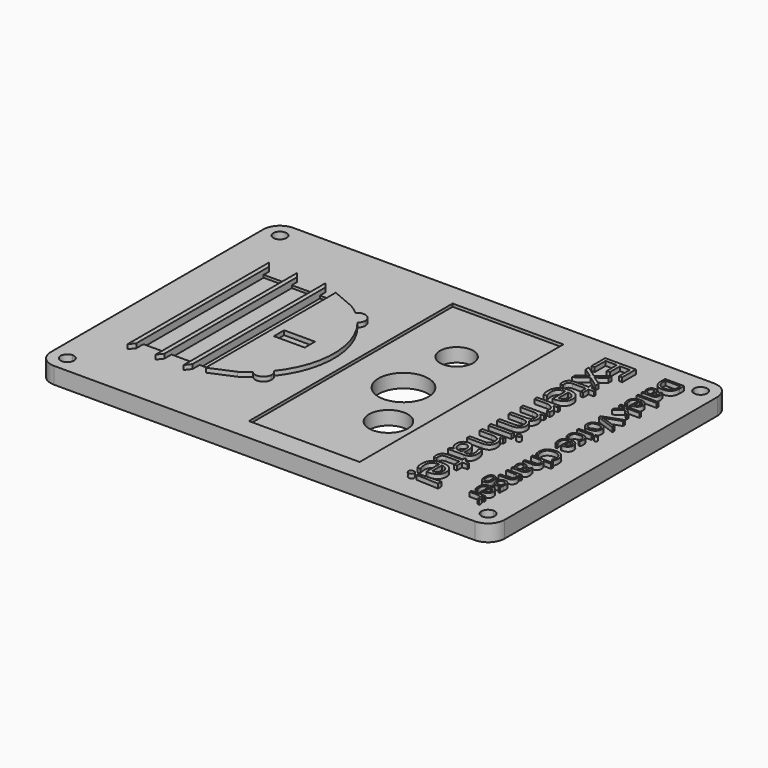
from build123d import *

# Parameters (mm, degrees)
F0_W           = 104.14
F0_H           = 68.58
F1_DEPTH       = 3.81
F2_R           = 3.81
F3_W           = 25.4
F3_H           = 58.42
F3_R           = 4.445
F3_R_2         = 5.715
F3_R_3         = 3.81
F4_DEPTH       = 0.66
F5_DEPTH       = 25.4
F3_W_2         = 7.0734824376
F3_H_2         = 2.9402009677
F3_TEXT_SIZE   = 9.8580958156
F3_TEXT_SIZE_2 = 6.0756268383
F6_DEPTH       = 1
F3_W_3         = 2.7178
F3_H_3         = 34.4777443152
F3_W_4         = 5.4356
F7_DEPTH       = 0.6


# Not quite as in the source:
# - Text() gives the source's letters only with a copy of the font that has no kerning and outlines rounded to 1/6400 em; it was checked with that copy


with BuildPart() as f1:
    # F0 (on Top) → F1 (new body)
    with BuildSketch(Plane.XY):
        with Locations((-0.150652461, 0.717826087)):
            Rectangle(F0_W, F0_H)
        with BuildLine():
            ThreePointArc((-48.410652461, 29.673826087), (-49.4882831955, 32.2754568215), (-46.886652461, 31.197826087))
            Line((-46.886652461, 31.197826087), (-44.600652461, 31.197826087))
            Line((-44.600652461, 31.197826087), (22.709347539, 31.197826087))
            Line((22.709347539, 31.197826087), (25.249347539, 31.197826087))
            Line((25.249347539, 31.197826087), (44.299347539, 31.197826087))
            Line((44.299347539, 31.197826087), (46.585347539, 31.197826087))
            ThreePointArc((46.585347539, 31.197826087), (48.109347539, 32.721826087), (49.633347539, 31.197826087))
            ThreePointArc((49.633347539, 31.197826087), (49.1869782735, 30.1201953524), (48.109347539, 29.673826087))
            Line((48.109347539, 29.673826087), (48.109347539, 27.387826087))
            Line((48.109347539, 27.387826087), (48.109347539, -25.952173913))
            Line((48.109347539, -25.952173913), (48.109347539, -28.238173913))
            ThreePointArc((48.109347539, -28.238173913), (49.1869782735, -28.6845431785), (49.633347539, -29.762173913))
            ThreePointArc((49.633347539, -29.762173913), (48.109347539, -31.286173913), (46.585347539, -29.762173913))
            Line((46.585347539, -29.762173913), (44.299347539, -29.762173913))
            Line((44.299347539, -29.762173913), (25.249347539, -29.762173913))
            Line((25.249347539, -29.762173913), (22.709347539, -29.762173913))
            Line((22.709347539, -29.762173913), (-44.600652461, -29.762173913))
            Line((-44.600652461, -29.762173913), (-46.886652461, -29.762173913))
            ThreePointArc((-46.886652461, -29.762173913), (-49.4882831955, -30.8398046476), (-48.410652461, -28.238173913))
            Line((-48.410652461, -28.238173913), (-48.410652461, -25.952173913))
            Line((-48.410652461, -25.952173913), (-48.410652461, 27.387826087))
            Line((-48.410652461, 27.387826087), (-48.410652461, 29.673826087))
        make_face(mode=Mode.SUBTRACT)
        Polygon((22.709347539, 31.197826087), (-44.600652461, 31.197826087), (-44.600652461, 27.387826087), (-48.410652461, 27.387826087), (-48.410652461, -25.952173913), (-44.600652461, -25.952173913), (-44.600652461, -29.762173913), (22.709347539, -29.762173913), (22.709347539, -24.682173913), (26.519347539, -20.872173913), (26.519347539, 15.957826087), (22.709347539, 19.767826087), align=None)
        Polygon((44.299347539, 31.197826087), (25.249347539, 31.197826087), (25.249347539, 19.767826087), (29.059347539, 15.957826087), (29.059347539, -20.872173913), (25.249347539, -24.682173913), (25.249347539, -29.762173913), (44.299347539, -29.762173913), (44.299347539, -25.952173913), (48.109347539, -25.952173913), (48.109347539, 27.387826087), (44.299347539, 27.387826087), align=None)
        Polygon((25.249347539, 31.197826087), (22.709347539, 31.197826087), (22.709347539, 19.767826087), (26.519347539, 15.957826087), (26.519347539, -20.872173913), (22.709347539, -24.682173913), (22.709347539, -29.762173913), (25.249347539, -29.762173913), (25.249347539, -24.682173913), (29.059347539, -20.872173913), (29.059347539, 15.957826087), (25.249347539, 19.767826087), align=None)
        with BuildLine():
            Line((-44.600652461, -25.952173913), (-48.410652461, -25.952173913))
            Line((-48.410652461, -25.952173913), (-48.410652461, -28.238173913))
            ThreePointArc((-48.410652461, -28.238173913), (-47.3330217265, -28.6845431785), (-46.886652461, -29.762173913))
            Line((-46.886652461, -29.762173913), (-44.600652461, -29.762173913))
            Line((-44.600652461, -29.762173913), (-44.600652461, -25.952173913))
        make_face()
        with BuildLine():
            Line((48.109347539, -28.238173913), (48.109347539, -25.952173913))
            Line((48.109347539, -25.952173913), (44.299347539, -25.952173913))
            Line((44.299347539, -25.952173913), (44.299347539, -29.762173913))
            Line((44.299347539, -29.762173913), (46.585347539, -29.762173913))
            ThreePointArc((46.585347539, -29.762173913), (47.0317168045, -28.6845431785), (48.109347539, -28.238173913))
        make_face()
        with BuildLine():
            Line((-44.600652461, 31.197826087), (-46.886652461, 31.197826087))
            ThreePointArc((-46.886652461, 31.197826087), (-47.3330217265, 30.1201953524), (-48.410652461, 29.673826087))
            Line((-48.410652461, 29.673826087), (-48.410652461, 27.387826087))
            Line((-48.410652461, 27.387826087), (-44.600652461, 27.387826087))
            Line((-44.600652461, 27.387826087), (-44.600652461, 31.197826087))
        make_face()
        with BuildLine():
            Line((46.585347539, 31.197826087), (44.299347539, 31.197826087))
            Line((44.299347539, 31.197826087), (44.299347539, 27.387826087))
            Line((44.299347539, 27.387826087), (48.109347539, 27.387826087))
            Line((48.109347539, 27.387826087), (48.109347539, 29.673826087))
            ThreePointArc((48.109347539, 29.673826087), (47.0317168045, 30.1201953524), (46.585347539, 31.197826087))
        make_face()
    extrude(amount=F1_DEPTH)

    # F2
    f2_edges = [f1.edges().sort_by_distance(p)[0] for p in [
        (-52.220652, -33.572174, 1.905),
        (-52.220652, 35.007826, 1.905),
        (51.919348, -33.572174, 1.905),
        (51.919348, 35.007826, 1.905),
    ]]
    fillet(f2_edges, radius=F2_R)

    # F3 (on face) → F4 (cut)
    with BuildSketch(Plane.XY.offset(3.81)):
        with Locations((4.929347539, 0.717826087)):
            Rectangle(F3_W, F3_H)
        with Locations((11.025347539, -11.982173913)):
            Circle(F3_R, mode=Mode.SUBTRACT)
        with Locations((4.929347539, -0.044173913)):
            Circle(F3_R_2, mode=Mode.SUBTRACT)
        with Locations((4.929347539, 15.195826087)):
            Circle(F3_R_3, mode=Mode.SUBTRACT)
        with Locations((4.929347539, -0.044173913)):
            Circle(F3_R_2)
        with Locations((11.025347539, -11.982173913)):
            Circle(F3_R)
    extrude(amount=-F4_DEPTH, mode=Mode.SUBTRACT)

    # F3 (on face) → F5 (cut)
    with BuildSketch(Plane.XY.offset(3.81)):
        with Locations((4.929347539, -0.044173913)):
            Circle(F3_R_2)
        with Locations((11.025347539, -11.982173913)):
            Circle(F3_R)
        with Locations((4.929347539, 15.195826087)):
            Circle(F3_R_3)
    extrude(amount=-F5_DEPTH, mode=Mode.SUBTRACT)

    # F3 (on face) → F6 (join)
    with BuildSketch(Plane.XY.offset(3.81)):
        Polygon((-28.268452461, -19.0365667301), (-28.268452461, -16.9964171946), (-28.268452461, 17.4813271206), (-28.268452461, 19.05), (-29.284452461, 20.32), (-29.284452461, 17.4813271206), (-29.284452461, -16.9964171946), (-29.284452461, -20.3065667301), align=None)
        Polygon((-34.720052461, -19.0365667301), (-34.720052461, -16.9964171946), (-34.720052461, 17.4813271206), (-34.720052461, 19.05), (-35.736052461, 20.32), (-35.736052461, 17.4813271206), (-35.736052461, -16.9964171946), (-35.736052461, -20.3065667301), align=None)
        Polygon((-41.171652461, -19.0365667301), (-41.171652461, -16.9964171946), (-41.171652461, 17.4813271206), (-41.171652461, 19.05), (-42.187652461, 20.32), (-42.187652461, -20.3065667301), align=None)
        with BuildLine():
            Line((-25.550652461, -18.6383566196), (-20.115052461, -16.3242976216))
            ThreePointArc((-20.115052461, -16.3242976216), (-18.9770344539, -15.5583765847), (-17.8965204495, -14.7132674168))
            ThreePointArc((-17.8965204495, -14.7132674168), (-17.8659765661, -12.086944828), (-15.2413653543, -11.9873493658))
            ThreePointArc((-15.2413653543, -11.9873493658), (-11.047252461, 0), (-15.2413653543, 11.9873493658))
            ThreePointArc((-15.2413653543, 11.9873493658), (-17.8659765661, 12.086944828), (-17.8965204495, 14.7132674168))
            ThreePointArc((-17.8965204495, 14.7132674168), (-18.9770344539, 15.5583765847), (-20.115052461, 16.3242976216))
            Line((-20.115052461, 16.3242976216), (-25.550652461, 18.6383566196))
            Line((-25.550652461, 18.6383566196), (-25.550652461, 17.4813271206))
            Line((-25.550652461, 17.4813271206), (-25.550652461, -16.9964171946))
            Line((-25.550652461, -16.9964171946), (-25.550652461, -18.6383566196))
        make_face()
        with Locations((-20.115052461, 0)):
            Rectangle(F3_W_2, F3_H_2, mode=Mode.SUBTRACT)
        with BuildLine():
            ThreePointArc((-17.8965204495, 14.7132674168), (-16.5013421202, 13.4161543032), (-15.2413653543, 11.9873493658))
            ThreePointArc((-15.2413653543, 11.9873493658), (-14.7650701457, 12.6323273896), (-14.5963421202, 13.4161543032))
            ThreePointArc((-14.5963421202, 13.4161543032), (-15.8044883756, 15.1891235242), (-17.8965204495, 14.7132674168))
        make_face()
        with BuildLine():
            ThreePointArc((-15.2413653543, -11.9873493658), (-16.5013421202, -13.4161543032), (-17.8965204495, -14.7132674168))
            ThreePointArc((-17.8965204495, -14.7132674168), (-15.8044883756, -15.1891235242), (-14.5963421202, -13.4161543032))
            ThreePointArc((-14.5963421202, -13.4161543032), (-14.7650701457, -12.6323273896), (-15.2413653543, -11.9873493658))
        make_face()
        with BuildLine():
            ThreePointArc((-15.2413653543, -11.9873493658), (-17.8659765661, -12.086944828), (-17.8965204495, -14.7132674168))
            ThreePointArc((-17.8965204495, -14.7132674168), (-16.5013421202, -13.4161543032), (-15.2413653543, -11.9873493658))
        make_face()
        with BuildLine():
            ThreePointArc((-17.8965204495, 14.7132674168), (-17.8659765661, 12.086944828), (-15.2413653543, 11.9873493658))
            ThreePointArc((-15.2413653543, 11.9873493658), (-16.5013421202, 13.4161543032), (-17.8965204495, 14.7132674168))
        make_face()
        with Locations(Location((28.0010672282, 29.927826087), (0, 0, -90))):
            Text('Exterminate!', F3_TEXT_SIZE, font='Open Sans', text_align=(TextAlign.LEFT, TextAlign.BOTTOM))
        with Locations(Location((41.4488962155, 29.927826087), (0, 0, -90))):
            Text('Dalek Voice Changer', F3_TEXT_SIZE_2, font='Open Sans', text_align=(TextAlign.LEFT, TextAlign.BOTTOM))
    extrude(amount=F6_DEPTH)

    # F3 (on face) → F7 (cut)
    with BuildSketch(Plane.XY.offset(3.81)):
        with Locations((-26.909552461, 0.242454963)):
            Rectangle(F3_W_3, F3_H_3)
        with Locations((-32.002252461, 0.242454963)):
            Rectangle(F3_W_4, F3_H_3)
        with Locations((-38.453852461, 0.242454963)):
            Rectangle(F3_W_4, F3_H_3)
    extrude(amount=-F7_DEPTH, mode=Mode.SUBTRACT)


solid = f1.part
